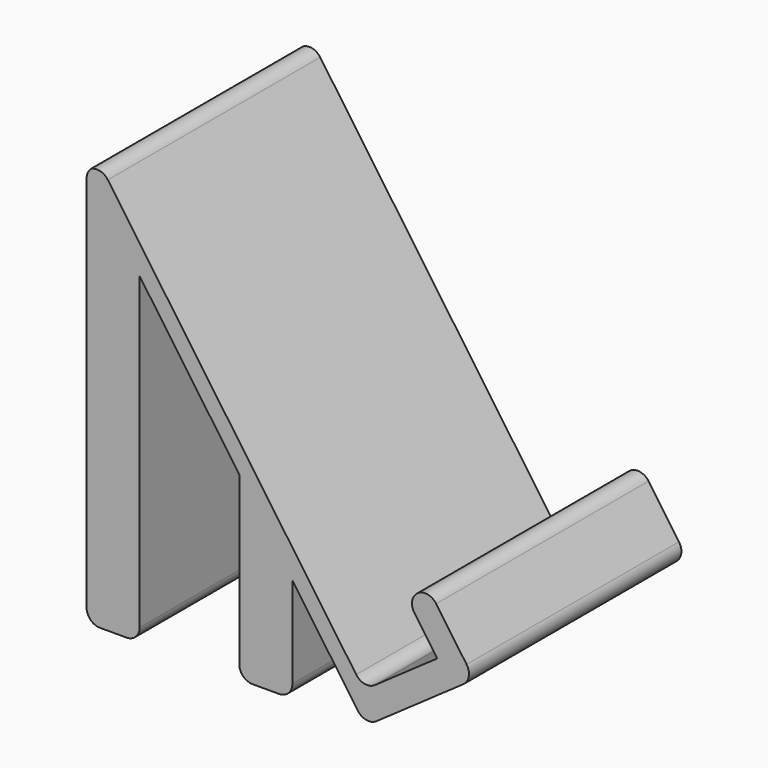
from build123d import *

# Parameters (mm, degrees)
F1_DEPTH    = 101.6
F3_DEPTH    = 6.35
F5_DEPTH    = 44.45
F6_W        = 10.16
F6_H        = 101.6
F7_DEPTH    = 20.32
F8_T1_DEPTH = 101.6
F8_T3_DEPTH = 127
F8_T5_DEPTH = 114.822403084
F10_W       = 251.0453239083
F10_H       = 203.9344906807
F11_DEPTH   = 160.782


# Not quite as in the source:
# - a fillet or chamfer that OpenCascade refuses, or shapes differently, is made with other operations: its cross-section is extruded or revolved along the edge and cut away or added


with BuildPart() as f1:
    # F0 (on Front) → F1 (new body)
    with BuildSketch(Plane.XZ):
        Polygon((57.3137016242, -18.4824153282), (36.9937016242, 10.5375521688), (36.9937016242, -58.4300412773), (57.3137016242, -58.4300412773), align=None)
    extrude(amount=F1_DEPTH)



with BuildPart() as f1b:
    # F0 (on Front) → F1, piece 2 (new body)
    with BuildSketch(Plane.XZ):
        Polygon((-1.1062983758, 64.9499912257), (-21.4262983758, 93.9699587227), (-21.4262983758, -58.4300412773), (-1.1062983758, -58.4300412773), align=None)
    extrude(amount=F1_DEPTH)


with BuildPart() as f1_1:
    add(f1.part)

    add(f1b.part)  # F3 merges F1b
    # F2 (on face) → F3 (join)
    with BuildSketch(Plane(origin=(29.774176385, 0, 20.8481027487), x_dir=(0, 1, 0), z_dir=(0.8191520443, 0, 0.5735764364))):
        Polygon((-101.6, 89.265303656), (-101.6, -96.780755544), (0, -96.780755544), (0, 38.465303656), (0, 89.265303656), align=None)
    extrude(amount=F3_DEPTH)

    # F4 (on face) → F5 (join)
    with BuildSketch(Plane(origin=(34.9757918662, 0, 24.4903131196), x_dir=(0, 1, 0), z_dir=(0.8191520443, 0, 0.5735764364))):
        Polygon((-101.6, -86.620755544), (-101.6, -96.780755544), (0, -96.780755544), (0, -86.620755544), (-12.7, -86.620755544), (-88.9, -86.620755544), align=None)
    extrude(amount=F5_DEPTH)

    # F6 (on face) → F7 (join)
    with BuildSketch(Plane(origin=(49.6836242789, 0, -70.9555689817), x_dir=(0.8191520443, 0, 0.5735764364), z_dir=(-0.5735764364, 0, 0.8191520443))):
        with Locations((82.0675579321, -50.8)):
            Rectangle(F6_W, F6_H)
    extrude(amount=F7_DEPTH)

    # F8: fillet of radius 5.08 on 11 edges, made by hand

    # F8_s2 → F8_t1 (join)
    with BuildSketch(Plane.XZ):
        with BuildLine():
            ThreePointArc((81.7456478485, -42.3039634771), (85.0248074909, -44.3930185658), (88.8207085301, -43.5514875655))
            Line((88.8207085301, -43.5514875655), (84.6594161452, -46.4652558621))
            Line((84.6594161452, -46.4652558621), (81.7456478485, -42.3039634771))
        make_face()
    extrude(amount=F8_T1_DEPTH)

    # F8_s4 → F8_t3 (cut)
    with BuildSketch(Plane.XZ.offset(-12.7)):
        with BuildLine():
            ThreePointArc((112.3294196238, -8.4859061114), (109.0502599814, -6.3968510227), (105.2543589422, -7.238382023))
            Line((105.2543589422, -7.238382023), (109.4156513272, -4.3246137264))
            Line((109.4156513272, -4.3246137264), (112.3294196238, -8.4859061114))
        make_face()
        with BuildLine():
            ThreePointArc((122.7369687221, -32.206136333), (124.8260238108, -28.9269766905), (123.9844928105, -25.1310756513))
            Line((123.9844928105, -25.1310756513), (126.8982611071, -29.2923680363))
            Line((126.8982611071, -29.2923680363), (122.7369687221, -32.206136333))
        make_face()
        with BuildLine():
            ThreePointArc((105.2543589422, -7.238382023), (103.1653038535, -10.5175416655), (104.0068348538, -14.3134427047))
            Line((104.0068348538, -14.3134427047), (101.0930665572, -10.1521503197))
            Line((101.0930665572, -10.1521503197), (105.2543589422, -7.238382023))
        make_face()
        with BuildLine():
            ThreePointArc((-13.3109145979, 93.4508767085), (-16.5900742404, 95.5399317971), (-20.3859752796, 94.6984007968))
            Line((-20.3859752796, 94.6984007968), (-16.2246828946, 97.6121690935))
            Line((-16.2246828946, 97.6121690935), (-13.3109145979, 93.4508767085))
        make_face()
        with BuildLine():
            ThreePointArc((82.3715689606, -54.2687586179), (85.650728603, -56.3578137066), (89.4466296422, -55.5162827063))
            Line((89.4466296422, -55.5162827063), (85.2853372573, -58.4300510029))
            Line((85.2853372573, -58.4300510029), (82.3715689606, -54.2687586179))
        make_face()
        with BuildLine():
            ThreePointArc((-16.3462983758, -58.4300412773), (-19.9384008243, -56.9421437258), (-21.4262983758, -53.3500412773))
            Line((-21.4262983758, -53.3500412773), (-21.4262983758, -58.4300412773))
            Line((-21.4262983758, -58.4300412773), (-16.3462983758, -58.4300412773))
        make_face()
        with BuildLine():
            ThreePointArc((-1.1062983758, -53.3500412773), (-2.5941959274, -56.9421437258), (-6.1862983758, -58.4300412773))
            Line((-6.1862983758, -58.4300412773), (-1.1062983758, -58.4300412773))
            Line((-1.1062983758, -58.4300412773), (-1.1062983758, -53.3500412773))
        make_face()
        with BuildLine():
            ThreePointArc((36.9937016242, -53.3500412773), (38.4815991757, -56.9421437258), (42.0737016242, -58.4300412773))
            Line((42.0737016242, -58.4300412773), (36.9937016242, -58.4300412773))
            Line((36.9937016242, -58.4300412773), (36.9937016242, -53.3500412773))
        make_face()
        with BuildLine():
            ThreePointArc((52.2337016242, -58.4300412773), (55.8258040726, -56.9421437258), (57.3137016242, -53.3500412773))
            Line((57.3137016242, -53.3500412773), (57.3137016242, -58.4300412773))
            Line((57.3137016242, -58.4300412773), (52.2337016242, -58.4300412773))
        make_face()
    extrude(amount=F8_T3_DEPTH, mode=Mode.SUBTRACT)

    # F8_s6 → F8_t5 (cut)
    with BuildSketch(Plane.XZ.offset(-6.611201542)):
        with BuildLine():
            ThreePointArc((-21.4262983758, 91.3254781059), (-20.8523134084, 93.6711610611), (-19.2600666725, 95.4867704908))
            Line((-19.2600666725, 95.4867704908), (-21.4262983758, 93.9699587227))
            Line((-21.4262983758, 93.9699587227), (-21.4262983758, 91.3254781059))
        make_face()
    extrude(amount=F8_T5_DEPTH, mode=Mode.SUBTRACT)


with BuildPart() as f9_1:
    # F9: copy of F1
    add(f1_1.part.moved(Location((0, 169.418, 0))))

    # F10 (on face) → F11 (cut)
    with BuildSketch(Plane.XZ.offset(-67.818)):
        with Locations((60.7606135309, 16.4267346263)):
            Rectangle(F10_W, F10_H)
    extrude(amount=-F11_DEPTH, mode=Mode.SUBTRACT)


solid = f1_1.part
